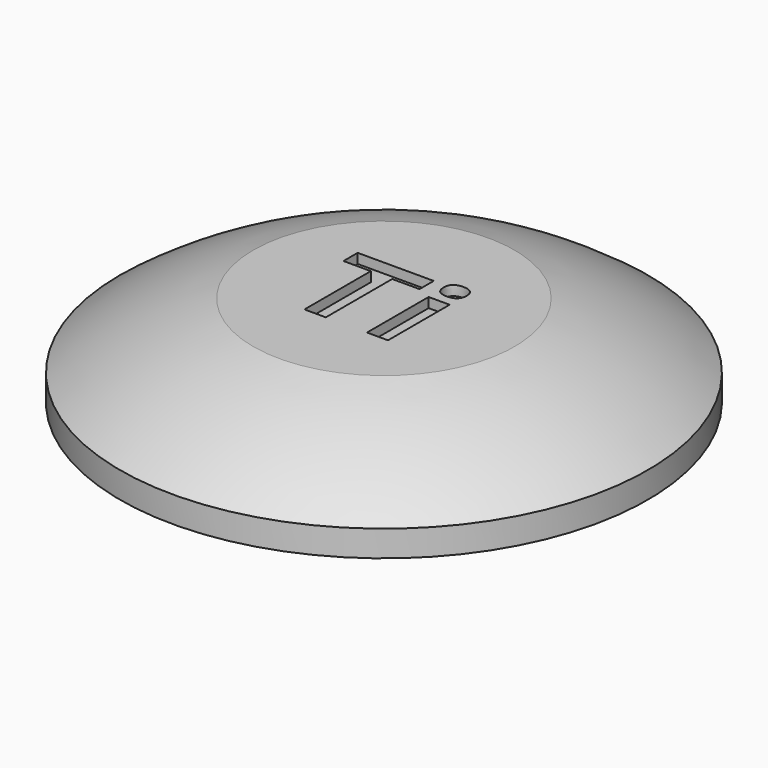
from build123d import *

# Parameters (mm, degrees)
F2_TEXT_SIZE = 21.5960466044
F3_DEPTH     = 1.5
F4_R         = 5
F5_SIZE      = 1


# Not quite as in the source:
# - Text() gives the source's letters only with a copy of the font that has no kerning and outlines rounded to 1/6400 em; it was checked with that copy


with BuildPart() as f1:
    # F0 (on Front) → F1 (revolve)
    with BuildSketch(Plane.XZ):
        with BuildLine():
            Line((-5.9, 0), (0, 0))
            Line((0, 0), (0, 14))
            Line((0, 14), (-20, 14))
            ThreePointArc((-20, 14), (-30.677634925, 9.974375247), (-40.4, 4))
            Line((-40.4, 4), (-40.4, 0))
            Line((-40.4, 0), (-20.4, 0))
            Line((-20.4, 0), (-20.4, 10))
            Line((-20.4, 10), (-5.9, 10))
            Line((-5.9, 10), (-5.9, 0))
        make_face()
    revolve(axis=Axis((0, 0, 7), (0, 0, 1)))

    # F2 (on face) → F3 (cut)
    with BuildSketch(Plane.XY.offset(14)):
        with Locations((-10.2502796799, -8.1654796377)):
            Text('Ti', F2_TEXT_SIZE, font='Open Sans', font_style=FontStyle.BOLD, text_align=(TextAlign.LEFT, TextAlign.BOTTOM))
    extrude(amount=-F3_DEPTH, mode=Mode.SUBTRACT)

    # F4
    f4_edges = [f1.edges().sort_by_distance(p)[0] for p in [
        (20.4, 0, 0),
    ]]
    fillet(f4_edges, radius=F4_R)

    # F5
    f5_edges = [f1.edges().sort_by_distance(p)[0] for p in [
        (5.9, 0, 0),
    ]]
    chamfer(f5_edges, length=F5_SIZE)


solid = f1.part
